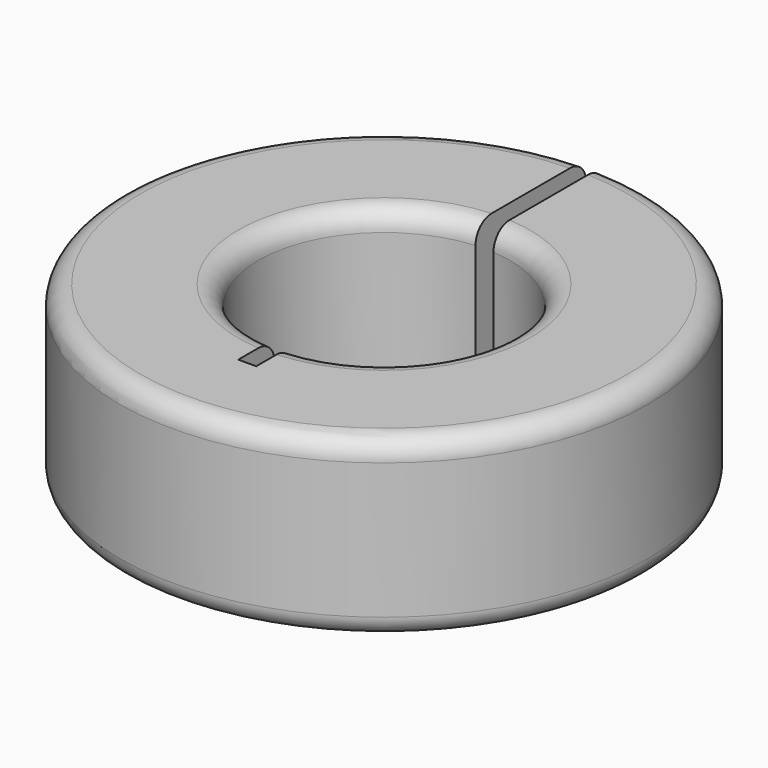
from build123d import *

# Parameters (mm, degrees)
F1_DEPTH = 11.1125
F2_R     = 1.27


# Not quite as in the source:
# - a feature names something its author has since deleted; it is built from what else it names


with BuildPart() as f1:
    # F0 (on Top) → F1 (new body)
    with BuildSketch(Plane.XY):
        with BuildLine():
            Line((0.5669642458, -7.9299578551), (0.5669642458, -10.7905164226))
            Line((0.5669642458, -10.7905164226), (-0.5669642458, -10.7905164226))
            Line((-0.5669642458, -10.7905164226), (-0.5669642458, -7.9299578551))
            ThreePointArc((-0.5669642458, -7.9299578551), (-7.950199987, -0.0004547511), (-0.5678714286, 7.9298929426))
            Line((-0.5678714286, 7.9298929426), (-0.5678714286, 16.659074062))
            ThreePointArc((-0.5678714286, 16.659074062), (0.0009076686, -16.6687499753), (0.5660571417, 16.6591358082))
            Line((0.5660571417, 16.6591358082), (0.5660571417, 7.9300226577))
            ThreePointArc((0.5660571417, 7.9300226577), (7.950199987, 0.0004547079), (0.5669642458, -7.9299578551))
        make_face()
    extrude(amount=F1_DEPTH)

    # F2
    f2_edges = [f1.edges().sort_by_distance(p)[0] for p in [
        (-7.9502, -0.000455, 11.1125),
        (-7.9502, -0.000455, 0),
        (0.000908, -16.66875, 11.1125),
        (0.000908, -16.66875, 0),
        (7.9502, 0.000455, 11.1125),
        (7.9502, 0.000455, 0),
    ]]
    fillet(f2_edges, radius=F2_R)


solid = f1.part
